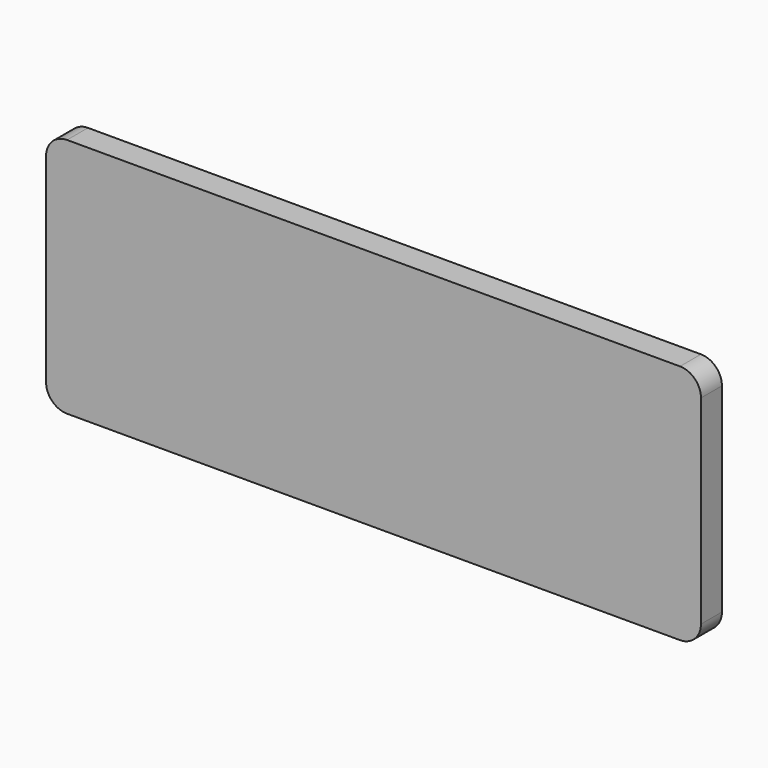
from build123d import *

# Parameters (mm, degrees)
F0_W     = 62.5
F0_H     = 23
F1_DEPTH = 2.5
F2_T     = -2
F3_R     = 2
F4_DEPTH = 2
F5_T     = -1.5
F6_R     = 2.5
F7_DEPTH = 2


# Not quite as in the source:
# - a feature names something its author has since deleted; it is built from what else it names


with BuildPart() as f1:
    # F0 (on Front) → F1 (new body)
    with BuildSketch(Plane.XZ):
        Rectangle(F0_W, F0_H)
    extrude(amount=F1_DEPTH)

    # F2
    f2_openings = [f1.faces().sort_by_distance(p)[0] for p in [
        (0, 0, 0),
    ]]
    offset(amount=F2_T, openings=f2_openings)

    # F3
    f3_edges = [f1.edges().sort_by_distance(p)[0] for p in [
        (-31.25, -1.25, 11.5),
        (-31.25, -1.25, -11.5),
        (31.25, -1.25, 11.5),
        (31.25, -1.25, -11.5),
    ]]
    fillet(f3_edges, radius=F3_R)

    # F4 (add): a face of the model
    f4_faces = [f1.faces().sort_by_distance(p)[0] for p in [
        (0, -0.5, 0),
    ]]
    extrude(f4_faces, amount=F4_DEPTH)

    # F5
    f5_openings = [f1.faces().sort_by_distance(p)[0] for p in [
        (0, 1.5, 0),
    ]]
    offset(amount=F5_T, openings=f5_openings, kind=Kind.INTERSECTION)

    # F6 (on face) → F7 (cut)
    with BuildSketch(Plane(origin=(0, 0, 0), x_dir=(-1, 0, 0), z_dir=(0, 1, 0))):
        with Locations((-28.75, 9)):
            Circle(F6_R)
        with Locations((28.75, 9)):
            Circle(F6_R)
        with Locations((28.75, -9)):
            Circle(F6_R)
        with Locations((-28.75, -9)):
            Circle(F6_R)
    extrude(amount=F7_DEPTH, mode=Mode.SUBTRACT)


solid = f1.part
